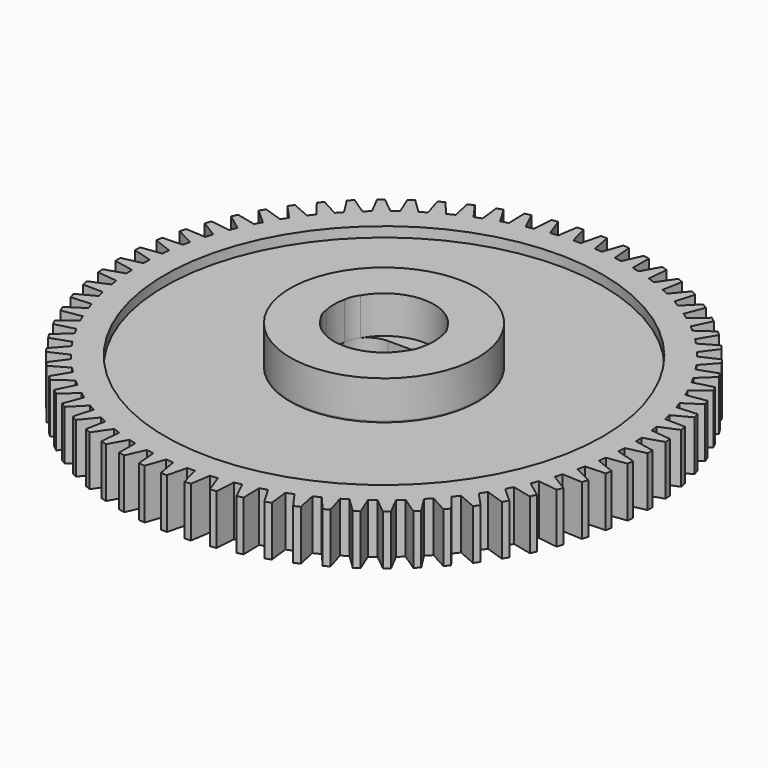
from build123d import *

# Parameters (mm, degrees)
F0_R     = 26.797
F0_R_2   = 22.225
F1_DEPTH = 2.54
F0_R_3   = 9.525
F2_DEPTH = 1.524
F3_DEPTH = 1.651
F4_R     = 9.525
F5_DEPTH = 3.81
F8_DEPTH = 5.081
F9_COUNT = 70


# Not quite as in the source:
# - a feature names something its author has since deleted; it is built from what else it names


with BuildPart() as f1:
    # F0 (on Top) → F1 (new body, symmetric)
    with BuildSketch(Plane.XY):
        Circle(F0_R)
        Circle(F0_R_2, mode=Mode.SUBTRACT)
    extrude(amount=F1_DEPTH, both=True)

    # F0 (on Top) → F2 (join, symmetric)
    with BuildSketch(Plane.XY):
        Circle(F0_R_2)
        Circle(F0_R_3, mode=Mode.SUBTRACT)
    extrude(amount=F2_DEPTH, both=True)

    # F0 (on Top) → F3 (join, symmetric)
    with BuildSketch(Plane.XY):
        Circle(F0_R_3)
        with BuildLine():
            ThreePointArc((4.953, -0.9525), (4.2090512242, -2.7485512242), (2.413, -3.4925))
            Line((2.413, -3.4925), (-2.413, -3.4925))
            ThreePointArc((-2.413, -3.4925), (-4.2090512242, -2.7485512242), (-4.953, -0.9525))
            Line((-4.953, -0.9525), (-4.953, 0.9525))
            ThreePointArc((-4.953, 0.9525), (-4.2090512242, 2.7485512242), (-2.413, 3.4925))
            Line((-2.413, 3.4925), (2.413, 3.4925))
            ThreePointArc((2.413, 3.4925), (4.2090512242, 2.7485512242), (4.953, 0.9525))
            Line((4.953, 0.9525), (4.953, -0.9525))
        make_face(mode=Mode.SUBTRACT)
    extrude(amount=F3_DEPTH, both=True)

    # F4 (on face) → F5 (join)
    with BuildSketch(Plane.XY.offset(1.651)):
        Circle(F4_R)
        with BuildLine():
            ThreePointArc((4.9438071766, 1.1684051526), (5.0458369205, 0.5881579477), (5.08, 0))
            ThreePointArc((5.08, 0), (5.0458369205, -0.5881579477), (4.9438071766, -1.1684051526))
            ThreePointArc((4.9438071766, -1.1684051526), (4.7755942622, -1.8851029982), (4.4089172093, -2.5234597365))
            ThreePointArc((4.4089172093, -2.5234597365), (0, -5.08), (-4.4089172093, -2.5234597365))
            ThreePointArc((-4.4089172093, -2.5234597365), (-4.7755942622, -1.8851029982), (-4.9438071766, -1.1684051526))
            ThreePointArc((-4.9438071766, -1.1684051526), (-5.08, 0), (-4.9438071766, 1.1684051526))
            ThreePointArc((-4.9438071766, 1.1684051526), (-4.7755942622, 1.8851029982), (-4.4089172093, 2.5234597365))
            ThreePointArc((-4.4089172093, 2.5234597365), (0, 5.08), (4.4089172093, 2.5234597365))
            ThreePointArc((4.4089172093, 2.5234597365), (4.7755942622, 1.8851029982), (4.9438071766, 1.1684051526))
        make_face(mode=Mode.SUBTRACT)
    extrude(amount=F5_DEPTH)

    # F6 (on face) → F8 (cut, through all)
    with BuildSketch(Plane.XY.offset(2.54)):
        with BuildLine():
            ThreePointArc((-1.793406814, 26.7369201854), (-2.6794264575, 26.6627058428), (-3.5624963012, 26.5591383351))
            Line((-3.5624963012, 26.5591383351), (-2.8603146919, 24.6523176861))
            Line((-2.8603146919, 24.6523176861), (-2.1021334831, 24.7285099076))
            Line((-2.1021334831, 24.7285099076), (-1.793406814, 26.7369201854))
        make_face()
        with BuildLine():
            Line((-2.7441904375, 27.3071657575), (-3.5624963012, 26.5591383351))
            ThreePointArc((-3.5624963012, 26.5591383351), (-2.6794264575, 26.6627058428), (-1.793406814, 26.7369201854))
            Line((-1.793406814, 26.7369201854), (-2.7441904375, 27.3071657575))
        make_face()
    f8 = extrude(amount=-F8_DEPTH, mode=Mode.SUBTRACT)

    # F9: F8 ×70 about axis
    f9_axis = Axis((0, 0, 8.8654514402), (0, 0, 1))
    for i in range(1, F9_COUNT):
        add(f8.rotate(f9_axis, i * 360 / F9_COUNT), mode=Mode.SUBTRACT)


solid = f1.part
